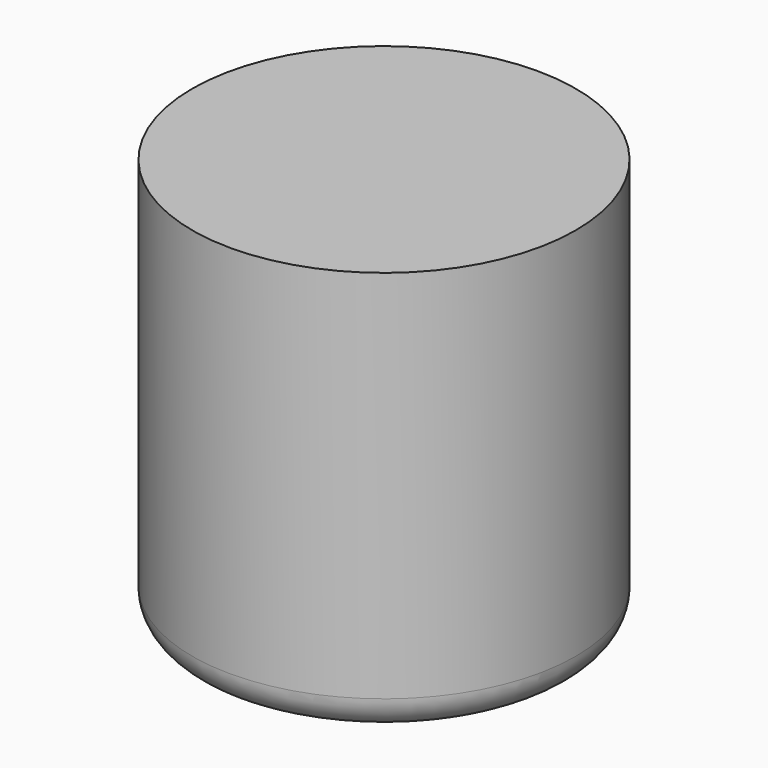
from build123d import *

# Parameters (mm, degrees)
F3_START = 0.7
F2_R     = 17.9818304379
F3_DEPTH = 38.3
F4_R     = 3.1384776311


# Not quite as in the source:
# - the program builds the solid bodies; features that only make, move or delete a surface that nothing else refers to are left out


with BuildPart() as f3:
    # F2 (on Top) → F3 (new body)
    with BuildSketch(Plane.XY.offset(F3_START)):
        Circle(F2_R)
    extrude(amount=F3_DEPTH)

    # F4
    f4_edges = [f3.edges().sort_by_distance(p)[0] for p in [
        (-17.98183, 0, 0.7),
    ]]
    fillet(f4_edges, radius=F4_R)


solid = f3.part
